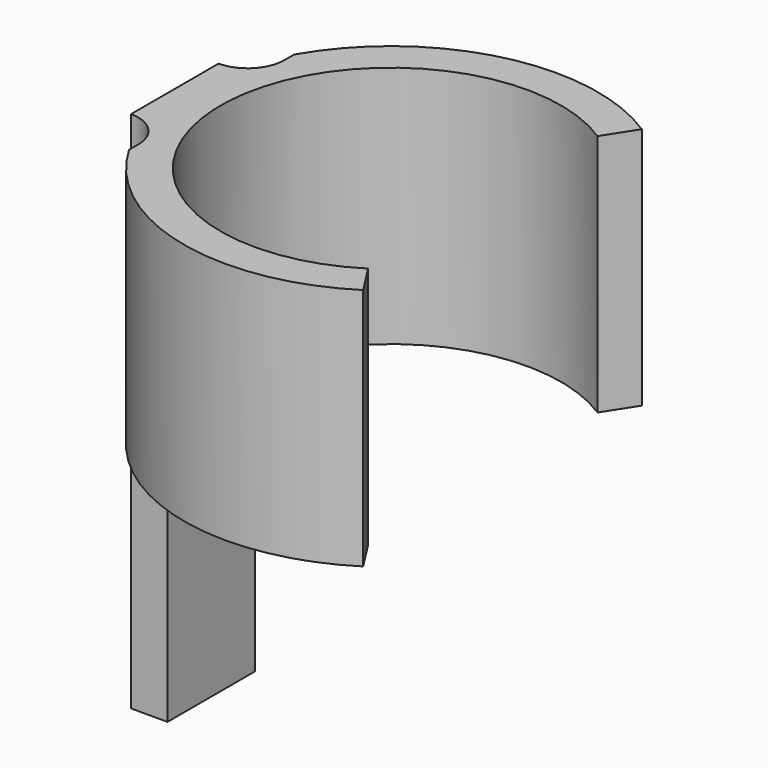
from build123d import *

# Parameters (mm, degrees)
F1_DEPTH = 20
F2_W     = 9
F2_H     = 43
F3_DEPTH = 3
F4_DEPTH = 3
F5_R     = 2.99999


# Not quite as in the source:
# - a fillet or chamfer is up to 0.001 mm smaller than in the source, because OpenCascade refuses the exact size
# - a feature names something its author has since deleted; it is built from what else it names


with BuildPart() as f1:
    # F0 (on Top) → F1 (new body)
    with BuildSketch(Plane.XY):
        with BuildLine():
            Line((7.553949271, 11.7871900982), (9.1726526862, 14.3130165478))
            ThreePointArc((9.1726526862, 14.3130165478), (-4.0313436719, 16.5150921341), (-14.7357025028, 8.4769730299))
            Line((-14.7357025028, 8.4769730299), (-14.7357025028, -8.4769730299))
            ThreePointArc((-14.7357025028, -8.4769730299), (-4.0313436719, -16.5150921341), (9.1726526862, -14.3130165478))
            Line((9.1726526862, -14.3130165478), (7.553949271, -11.7871900982))
            ThreePointArc((7.553949271, -11.7871900982), (-14, 0), (7.553949271, 11.7871900982))
        make_face()
    extrude(amount=F1_DEPTH)

    # F2 (on face) → F3 (join)
    with BuildSketch(Plane(origin=(-14.7357025028, 0, 0), x_dir=(0, -1, 0), z_dir=(-1, 0, 0))):
        with Locations((0.0303052693, -1.5)):
            Rectangle(F2_W, F2_H)
    extrude(amount=F3_DEPTH)

    # F2 (on face) → F4 (join)
    with BuildSketch(Plane(origin=(-14.7357025028, 0, 0), x_dir=(0, -1, 0), z_dir=(-1, 0, 0))):
        with Locations((0.0303052693, -1.5)):
            Rectangle(F2_W, F2_H)
    extrude(amount=F4_DEPTH)

    # F5 (radius 3 in the source; OpenCascade refuses exactly that, so slightly less here)
    f5_edges = [f1.edges().sort_by_distance(p)[0] for p in [
        (-14.735703, 4.469695, 10),
        (-14.735703, -4.530305, 10),
    ]]
    fillet(f5_edges, radius=F5_R)


solid = f1.part
